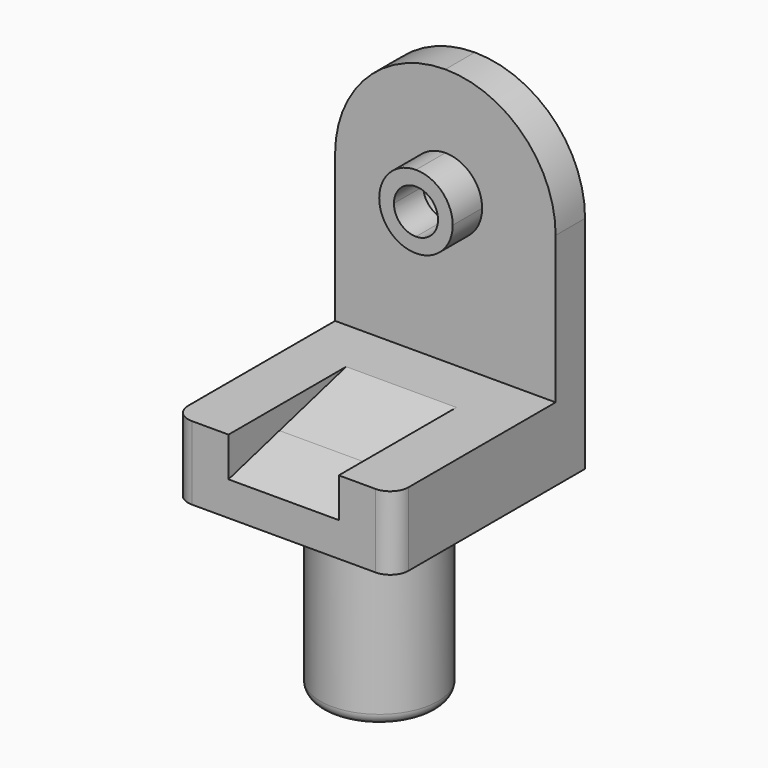
from build123d import *

# Parameters (mm, degrees)
F0_R      = 16
F1_DEPTH  = 50
F3_DEPTH  = 20
F4_DEPTH  = 20
F6_DEPTH  = 30
F7_DEPTH  = 40
F8_W      = 60
F8_H      = 10
F9_DEPTH  = 70
F10_R     = 29.99999
F11_R     = 3
F12_R     = 5
F14_D     = 17
F15_DEPTH = 10


# Not quite as in the source:
# - a fillet or chamfer is up to 0.001 mm smaller than in the source, because OpenCascade refuses the exact size


with BuildPart() as f1:
    # F0 (on Top) → F1 (new body)
    with BuildSketch(Plane.XY):
        Circle(F0_R)
    extrude(amount=F1_DEPTH)

    # F2 (on face) → F3 (join)
    with BuildSketch(Plane.XY.offset(50)):
        with BuildLine():
            Line((-30, 32.5), (-30, 7.5))
            Line((-30, 7.5), (-14.1332940251, 7.5))
            ThreePointArc((-14.1332940251, 7.5), (0, 16), (14.1332940251, 7.5))
            Line((14.1332940251, 7.5), (15, 7.5))
            Line((15, 7.5), (30, 7.5))
            Line((30, 7.5), (30, 32.5))
            Line((30, 32.5), (0, 32.5))
            Line((0, 32.5), (-30, 32.5))
        make_face()
        with BuildLine():
            ThreePointArc((14.1332940251, 7.5), (0, 16), (-14.1332940251, 7.5))
            Line((-14.1332940251, 7.5), (14.1332940251, 7.5))
        make_face()
    extrude(amount=F3_DEPTH)

    # F2 (on face) → F4 (join)
    with BuildSketch(Plane.XY.offset(50)):
        with BuildLine():
            Line((15, 5.5677643628), (15, -5.5677643628))
            ThreePointArc((15, -5.5677643628), (15.748015748, -2.8284271247), (16, 0))
            ThreePointArc((16, 0), (15.748015748, 2.8284271247), (15, 5.5677643628))
        make_face()
        with BuildLine():
            ThreePointArc((16, 0), (15.748015748, -2.8284271247), (15, -5.5677643628))
            Line((15, -5.5677643628), (15, -32.5))
            Line((15, -32.5), (30, -32.5))
            Line((30, -32.5), (30, 0))
            Line((30, 0), (30, 7.5))
            Line((30, 7.5), (15, 7.5))
            Line((15, 7.5), (15, 5.5677643628))
            ThreePointArc((15, 5.5677643628), (15.748015748, 2.8284271247), (16, 0))
        make_face()
    extrude(amount=F4_DEPTH)

    # F5 (on face) → F6 (join)
    with BuildSketch(Plane(origin=(15, 0, 0), x_dir=(0, -1, 0), z_dir=(-1, 0, 0))):
        Polygon((3.8423609018, 66.9608235561), (-7.5, 70), (-7.5, 50), (-5.5677643628, 50), (5.5677643628, 50), (32.5, 50), (32.5, 59.2820323028), (15.1847218036, 63.9216471122), align=None)
    extrude(amount=F6_DEPTH)

    # F7 (add): a face of the model
    f7_faces = [f1.faces().sort_by_distance(p)[0] for p in [
        (-22.5, 7.5, 60),
    ]]
    extrude(f7_faces, amount=F7_DEPTH)

    # F8 (on face) → F9 (join)
    with BuildSketch(Plane.XY.offset(70)):
        with Locations((0, 27.5)):
            Rectangle(F8_W, F8_H)
    extrude(amount=F9_DEPTH)

    # F10 (radius 30 in the source; OpenCascade refuses exactly that, so slightly less here)
    f10_edges = [f1.edges().sort_by_distance(p)[0] for p in [
        (-30, 27.5, 140),
        (30, 27.5, 140),
    ]]
    fillet(f10_edges, radius=F10_R)

    # F11
    f11_edges = [f1.edges().sort_by_distance(p)[0] for p in [
        (-16, 0, 0),
    ]]
    fillet(f11_edges, radius=F11_R)

    # F12
    f12_edges = [f1.edges().sort_by_distance(p)[0] for p in [
        (-30, -32.5, 60),
        (30, -32.5, 60),
    ]]
    fillet(f12_edges, radius=F12_R)

    # F14 (through all)
    with Locations(Plane.XZ.offset(-22.5)):
        with Locations((0, 110)):
            Hole(F14_D / 2)

    # F13 (on face) → F15 (join)
    with BuildSketch(Plane.XZ.offset(-22.5)):
        with BuildLine():
            Line((-6, 110), (-10, 110))
            ThreePointArc((-10, 110), (-7.0710678119, 102.9289321881), (0, 100))
            Line((0, 100), (0, 104))
            ThreePointArc((0, 104), (-4.2426406871, 105.7573593129), (-6, 110))
        make_face()
        with BuildLine():
            Line((0, 116), (0, 120))
            ThreePointArc((0, 120), (-7.0710678119, 117.0710678119), (-10, 110))
            Line((-10, 110), (-6, 110))
            ThreePointArc((-6, 110), (-4.2426406871, 114.2426406871), (0, 116))
        make_face()
        with BuildLine():
            ThreePointArc((10, 110), (7.0710678119, 117.0710678119), (0, 120))
            Line((0, 120), (0, 116))
            ThreePointArc((0, 116), (4.2426406871, 114.2426406871), (6, 110))
            Line((6, 110), (10, 110))
        make_face()
        with BuildLine():
            ThreePointArc((0, 100), (7.0710678119, 102.9289321881), (10, 110))
            Line((10, 110), (6, 110))
            ThreePointArc((6, 110), (4.2426406871, 105.7573593129), (0, 104))
            Line((0, 104), (0, 100))
        make_face()
    extrude(amount=F15_DEPTH)


solid = f1.part
